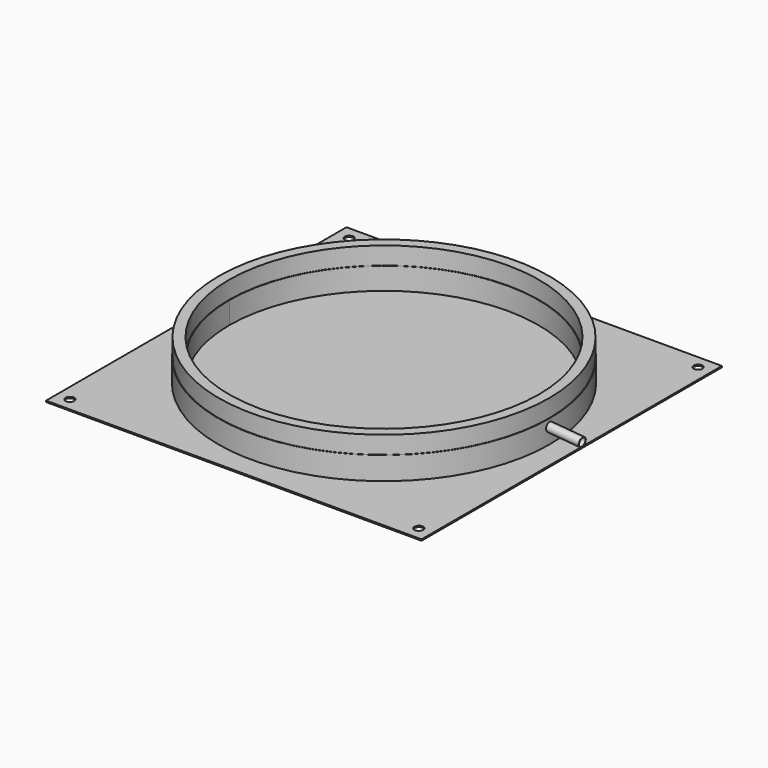
from build123d import *
from build123d import SkipClean  # not in build123d's __all__

# Parameters (mm, degrees)
F0_W     = 10
F0_H     = 3
F2_W     = 850
F2_H     = 850
F2_R     = 10
F3_DEPTH = 3
F6_R     = 9
F7_DEPTH = 120
F8_R     = 350
F9_DEPTH = 200


with BuildPart() as f1:
    # F0 (on Front) → F1 (revolve)
    with BuildSketch(Plane.XZ):
        Polygon((-375, 5), (-350, 5), (-350, 55), (-351, 55), (-351, 95), (-374, 95), (-374, 55), (-375, 55), align=None)
        Polygon((-10, 5), (-350, 5), (-375, 5), (-375, 2), (-10, 2), align=None)
        with Locations((-5, 3.5)):
            Rectangle(F0_W, F0_H)
    revolve(axis=Axis((0, 0, 187.9212413023), (0, 0, -1)))

    # F2 (on Top) → F3 (join)
    with BuildSketch(Plane.XY):
        Rectangle(F2_W, F2_H)
        with Locations((-395, -395)):
            Circle(F2_R, mode=Mode.SUBTRACT)
        with Locations((395, -395)):
            Circle(F2_R, mode=Mode.SUBTRACT)
        with Locations((-395, 395)):
            Circle(F2_R, mode=Mode.SUBTRACT)
        with Locations((395, 395)):
            Circle(F2_R, mode=Mode.SUBTRACT)
    extrude(amount=F3_DEPTH)

    # F4 (on Front) → F5 (revolve)
    with BuildSketch(Plane.XZ):
        Polygon((449.6194698092, 41.5098406888), (350, 50.2254149636), (349.9128442573, 49.2292202655), (449.5323140664, 40.5136459907), align=None)
    revolve(axis=Axis((462.7442754949, 0, 30.3233706049), (0.9961946981, 0, -0.0871557427)))

    # F6 (on face) → F7 (cut)
    with BuildSketch(Plane(origin=(442.6000506958, 0, -38.7224869119), x_dir=(0, 1, 0), z_dir=(0.9961946981, 0, -0.0871557427))):
        with Locations((0, 70.5388020579)):
            Circle(F6_R)
    extrude(amount=-F7_DEPTH, mode=Mode.SUBTRACT)

    # F8 (on face) → F9 (cut)
    with BuildSketch(Plane.XY.offset(5)):
        Circle(F8_R)
    with SkipClean():  # cleaning this boolean's faces spoils the solid; the shape is the same uncleaned
        extrude(amount=F9_DEPTH, mode=Mode.SUBTRACT)


solid = f1.part
